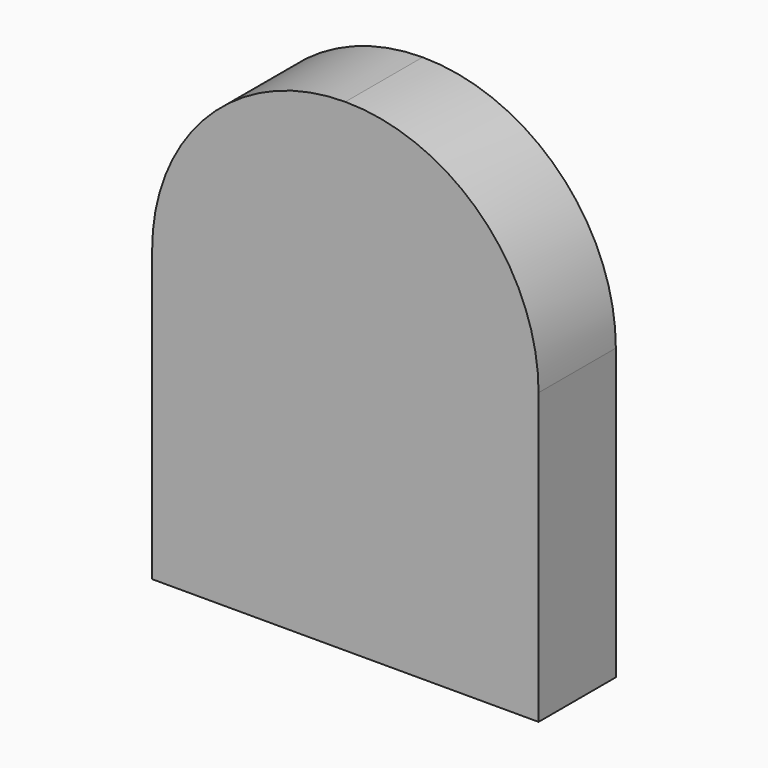
from build123d import *

# Parameters (mm, degrees)
F0_W     = 101.6
F0_H     = 127
F1_DEPTH = 25.4
F2_R     = 50.79999


# Not quite as in the source:
# - a fillet or chamfer is up to 0.001 mm smaller than in the source, because OpenCascade refuses the exact size


with BuildPart() as f1:
    # F0 (on Front) → F1 (new body)
    with BuildSketch(Plane.XZ):
        with Locations((11.2417165004, 3.3230111003)):
            Rectangle(F0_W, F0_H)
    extrude(amount=F1_DEPTH)

    # F2 (radius 50.8 in the source; OpenCascade refuses exactly that, so slightly less here)
    f2_edges = [f1.edges().sort_by_distance(p)[0] for p in [
        (62.041717, -12.7, 66.823011),
        (-39.558283, -12.7, 66.823011),
    ]]
    fillet(f2_edges, radius=F2_R)


solid = f1.part
